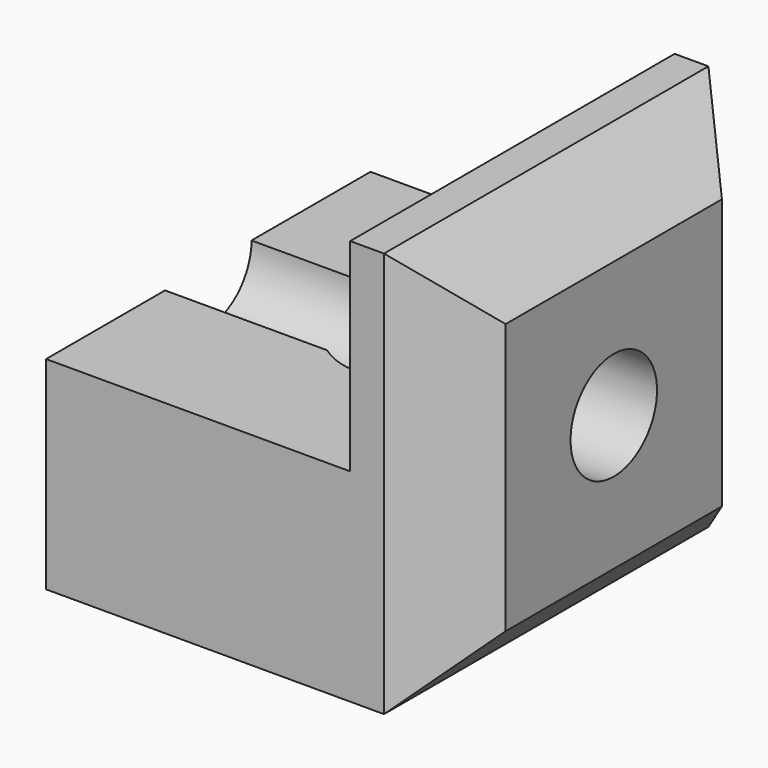
from build123d import *

# Parameters (mm, degrees)
F0_W     = 30
F0_H     = 30
F1_DEPTH = 30
F2_R     = 4
F3_DEPTH = 30.001
F4_R     = 5
F5_DEPTH = 30.001
F6_W     = 30
F6_H     = 15
F7_DEPTH = 22.5
F8_SIZE  = 5
F9_SIZE  = 4.99999


# Not quite as in the source:
# - a fillet or chamfer is up to 0.001 mm smaller than in the source, because OpenCascade refuses the exact size


with BuildPart() as f1:
    # F0 (on Top) → F1 (new body)
    with BuildSketch(Plane.XY):
        with Locations((0.4279911518, -7.855784721)):
            Rectangle(F0_W, F0_H)
    extrude(amount=F1_DEPTH)

    # F2 (on face) → F3 (cut, through all)
    with BuildSketch(Plane(origin=(-14.5720088482, 0, 0), x_dir=(0, -1, 0), z_dir=(-1, 0, 0))):
        with Locations((7.855784721, 15)):
            Circle(F2_R)
    extrude(amount=-F3_DEPTH, mode=Mode.SUBTRACT)

    # F4 (on face) → F5 (cut, through all)
    with BuildSketch(Plane.XY.offset(30)):
        with Locations((0.4279911518, -7.855784721)):
            Circle(F4_R)
    extrude(amount=-F5_DEPTH, mode=Mode.SUBTRACT)

    # F6 (on face) → F7 (cut)
    with BuildSketch(Plane(origin=(-14.5720088482, 0, 0), x_dir=(0, -1, 0), z_dir=(-1, 0, 0))):
        with Locations((7.855784721, 22.5)):
            Rectangle(F6_W, F6_H)
    extrude(amount=-F7_DEPTH, mode=Mode.SUBTRACT)

    # F8
    f8_edges = [f1.edges().sort_by_distance(p)[0] for p in [
        (-4.572009, -7.855785, 0),
    ]]
    chamfer(f8_edges, length=F8_SIZE)

    # F9 (size 5 in the source; OpenCascade refuses exactly that, so slightly less here)
    f9_edges = [f1.edges().sort_by_distance(p)[0] for p in [
        (15.427991, -7.855785, 30),
        (15.427991, -22.855785, 15),
        (15.427991, 7.144215, 15),
        (15.427991, -7.855785, 0),
    ]]
    chamfer(f9_edges, length=F9_SIZE)


solid = f1.part
